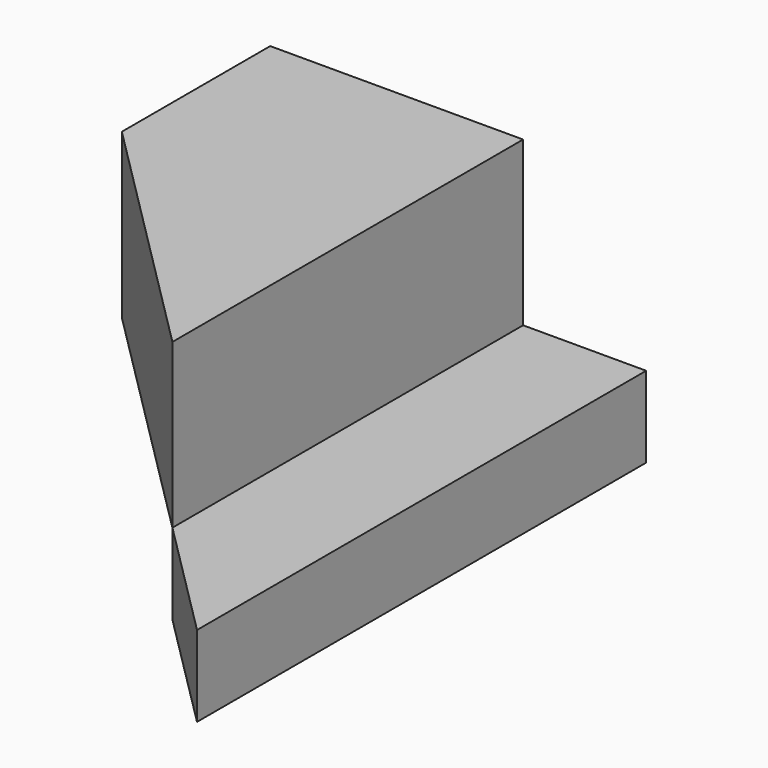
from build123d import *

# Parameters (mm, degrees)
F1_W        = 463.55
F1_H        = 304.8
F2_DEPTH    = 2120.9
F1_W_2      = 952.5
F1_H_2      = 615.95
F3_DEPTH    = 1651
F4_T1_DEPTH = 2721.6676720904
F5_SIZE     = 952.49999


# Not quite as in the source:
# - a fillet or chamfer that OpenCascade refuses, or shapes differently, is made with other operations: its cross-section is extruded or revolved along the edge and cut away or added
# - a fillet or chamfer is up to 0.001 mm smaller than in the source, because OpenCascade refuses the exact size


with BuildPart() as f2:
    # F1 (on face) → F2 (new body)
    with BuildSketch(Plane.XZ):
        with Locations((6.0013753094, 19.2331727594)):
            Rectangle(F1_W, F1_H)
    extrude(amount=F2_DEPTH)

    # F4: chamfer of 469.9 on 1 edges, made by hand

    # F4_s2 → F4_t1 (cut)
    with BuildSketch(Plane.XY.offset(-1341.6006632858)):
        Polygon((-225.7736246906, -1651), (244.1263753094, -2120.9), (-225.7736246906, -2120.9), align=None)
    extrude(amount=F4_T1_DEPTH, mode=Mode.SUBTRACT)


with BuildPart() as f3:
    # F1 (on face) → F3 (new body)
    with BuildSketch(Plane.XZ):
        with Locations((-702.0236246906, 479.6081727594)):
            Rectangle(F1_W_2, F1_H_2)
    extrude(amount=F3_DEPTH)

    # F5 (size 952.5 in the source; OpenCascade refuses exactly that, so slightly less here)
    f5_edges = [f3.edges().sort_by_distance(p)[0] for p in [
        (-1178.273625, -1651, 479.608173),
    ]]
    chamfer(f5_edges, length=F5_SIZE)


solid = Compound([f2.part, f3.part])
